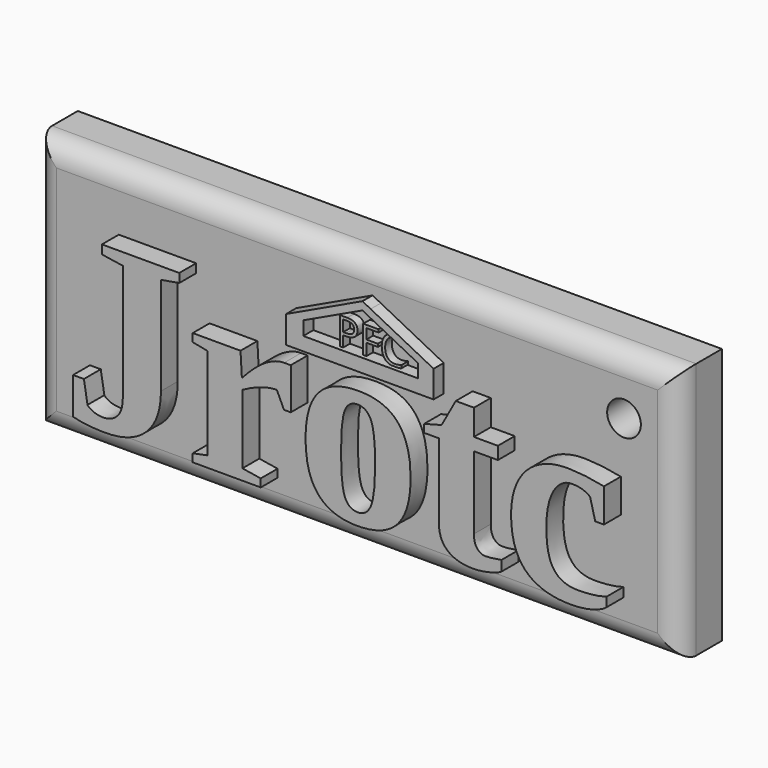
from build123d import *

# Parameters (mm, degrees)
F0_W         = 152.9011279345
F0_H         = 60.9747394919
F1_DEPTH     = 12.7
F2_R         = 5.08
F3_TEXT_SIZE = 58.8450296265
F4_DEPTH     = 5
F5_W         = 27.1757308985
F5_H         = 3.2087567068
F6_DEPTH     = 3
F7_TEXT_SIZE = 9.1600492464
F8_DEPTH     = 2
F9_R         = 4
F10_DEPTH    = 12.701


# Not quite as in the source:
# - Text() gives the source's letters only with a copy of the font that has no kerning and outlines rounded to 1/6400 em; it was checked with that copy


with BuildPart() as f1:
    # F0 (on Front) → F1 (new body)
    with BuildSketch(Plane.XZ):
        Rectangle(F0_W, F0_H)
    extrude(amount=F1_DEPTH)

    # F2
    f2_edges = [f1.edges().sort_by_distance(p)[0] for p in [
        (0, -12.7, 30.48737),
        (-76.450564, -12.7, 0),
        (0, -12.7, -30.48737),
        (76.450564, -12.7, 0),
    ]]
    fillet(f2_edges, radius=F2_R)

    # F3 (on face) → F4 (join)
    with BuildSketch(Plane.XZ.offset(12.7)):
        with Locations((-66.0087764263, -22.2587715834)):
            Text('Jrotc', F3_TEXT_SIZE, font='Tinos', font_style=FontStyle.BOLD, text_align=(TextAlign.LEFT, TextAlign.BOTTOM))
    extrude(amount=F4_DEPTH)

    # F5 (on face) → F6 (join)
    with BuildSketch(Plane.XZ.offset(12.7)):
        Polygon((-14.4298253581, 12.7000900523), (-14.4298253581, 8.135965094), (-10.3651381002, 8.135965094), (-10.3651381002, 11.3447218008), (-10.3651381002, 14.6207074069), align=None)
        with Locations((3.2227273491, 9.7403434474)):
            Rectangle(F5_W, F5_H)
        Polygon((-14.4298253581, 14.6207074069), (-14.4298253581, 12.7000900523), (-10.3651381002, 14.6207074069), (3.6842117552, 21.2592071094), (5.6373054475, 22.1820691656), (3.6842117552, 23.179824464), align=None)
        Polygon((16.8105927984, 11.3447218008), (16.8105927984, 8.135965094), (20.5701775849, 8.135965094), (20.5701775849, 12.632861153), (16.8105927984, 14.5534785075), align=None)
        Polygon((5.6373054475, 22.1820691656), (3.6842117552, 21.2592071094), (16.8105927984, 14.5534785075), (20.5701775849, 12.632861153), (20.5701775849, 14.5534785075), align=None)
    extrude(amount=F6_DEPTH)

    # F7 (on face) → F8 (join)
    with BuildSketch(Plane.XZ.offset(12.7)):
        with Locations((-3.3404631725, 11.3447218008)):
            Text('PFC', F7_TEXT_SIZE, font='Open Sans', text_align=(TextAlign.LEFT, TextAlign.BOTTOM))
    extrude(amount=F8_DEPTH)

    # F9 (on face) → F10 (cut, through all)
    with BuildSketch(Plane.XZ.offset(12.7)):
        with Locations((63.3705639672, 16.8733976151)):
            Circle(F9_R)
    extrude(amount=-F10_DEPTH, mode=Mode.SUBTRACT)


solid = f1.part
